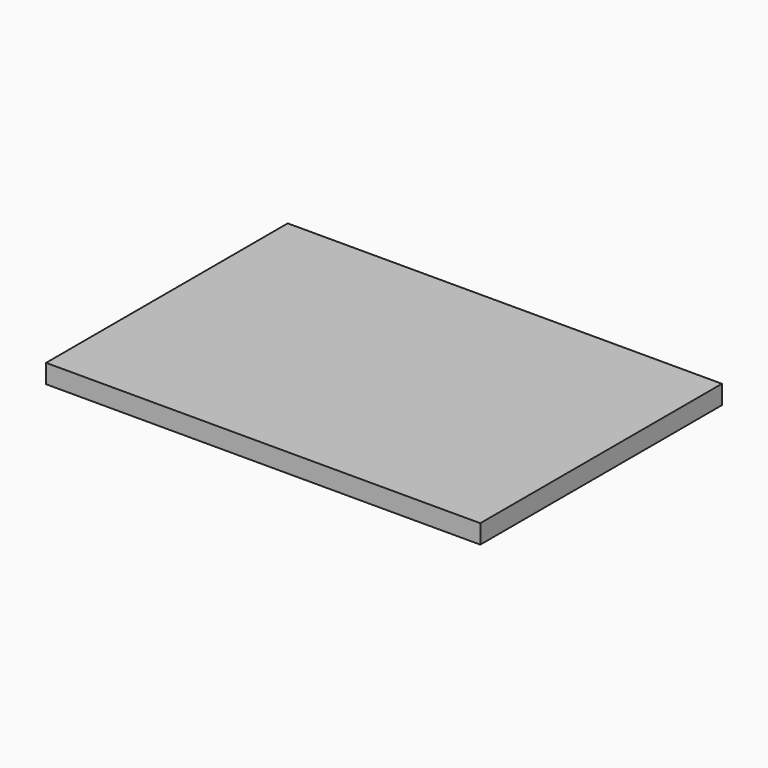
from build123d import *

# Parameters (mm, degrees)
F0_W     = 230
F0_H     = 160
F1_DEPTH = 10


# Not quite as in the source:
# - a feature names something its author has since deleted; it is built from what else it names


with BuildPart() as f1:
    # F0 (on Top) → F1 (new body)
    with BuildSketch(Plane.XY):
        Rectangle(F0_W, F0_H)
    extrude(amount=F1_DEPTH)


solid = f1.part
